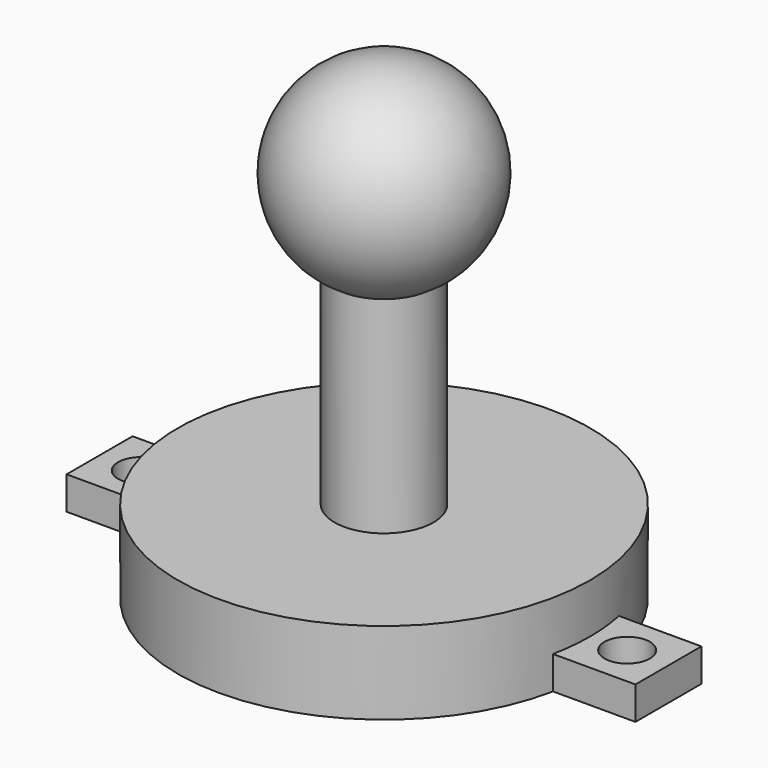
from build123d import *

# Parameters (mm, degrees)
F2_W     = 10
F2_H     = 10
F2_R     = 2.75
F3_DEPTH = 4


# Not quite as in the source:
# - a pattern or mirror of a feature is missing from the dataset's text; its kind, count and spacing are read off the source's solid


with BuildPart() as f1:
    # F0 (on Front) → F1 (revolve)
    with BuildSketch(Plane.XZ):
        with BuildLine():
            Line((25, 10), (6, 10))
            Line((6, 10), (6, 35))
            ThreePointArc((6, 35), (11.5911099155, 48.4981333866), (0, 57.3923048454))
            Line((0, 57.3923048454), (0, 0))
            Line((0, 0), (25, 0))
            Line((25, 0), (25, 10))
        make_face()
    revolve(axis=Axis((0, 0, 28.6961524227), (0, 0, -1)))

    # F2 (on face) → F3 (join)
    with BuildSketch(Plane(origin=(0, 0, 0), x_dir=(1, 0, 0), z_dir=(0, 0, -1))):
        with Locations((29.4948974278, 0)):
            Rectangle(F2_W, F2_H)
        with Locations((29.4948974278, 0)):
            Circle(F2_R, mode=Mode.SUBTRACT)
    f3 = extrude(amount=-F3_DEPTH)

    # F3_copies: F3 across plane
    add(f3.mirror(Plane(origin=(0, 0, 0), x_dir=(0, 0, -1), z_dir=(-1, 0, 0))))


solid = f1.part
